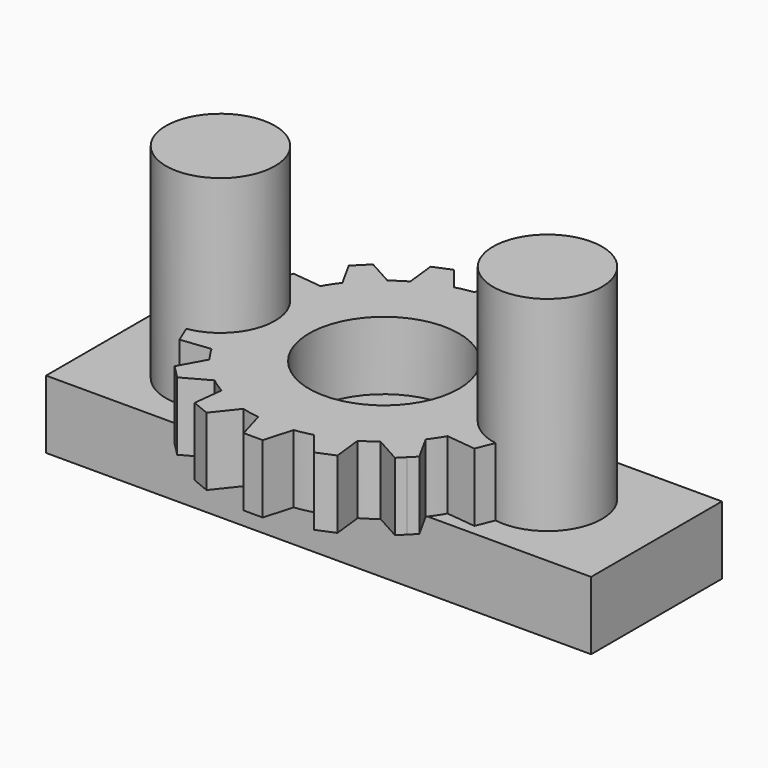
from build123d import *

# Parameters (mm, degrees)
F0_R     = 27.5
F1_DEPTH = 25
F2_W     = 200
F2_H     = 60
F2_R     = 20
F3_DEPTH = 25
F4_DEPTH = 75


with BuildPart() as f1:
    # F0 (on Top) → F1 (new body)
    with BuildSketch(Plane.XY):
        with BuildLine():
            ThreePointArc((-24.9770158815, 43.3145319454), (-19.1341716183, 46.1939766256), (-12.9665819589, 48.2894165662))
            Line((-12.9665819589, 48.2894165662), (-19.7274275781, 56.772163964))
            Line((-19.7274275781, 56.772163964), (-22.9610059419, 55.4327719507))
            Line((-22.9610059419, 55.4327719507), (-26.1945843057, 54.0933799374))
            Line((-26.1945843057, 54.0933799374), (-24.9770158815, 43.3145319454))
        make_face()
        with BuildLine():
            ThreePointArc((-39.6515075123, 30.4591193569), (-35.3553390593, 35.3553390593), (-30.4591193569, 39.6515075123))
            Line((-30.4591193569, 39.6515075123), (-39.951533137, 44.9012806053))
            Line((-39.951533137, 44.9012806053), (-42.4264068712, 42.4264068712))
            Line((-42.4264068712, 42.4264068712), (-44.9012806053, 39.951533137))
            Line((-44.9012806053, 39.951533137), (-39.6515075123, 30.4591193569))
        make_face()
        with BuildLine():
            ThreePointArc((-48.2894165662, 12.9665819589), (-46.1939766256, 19.1341716183), (-43.3145319454, 24.9770158815))
            Line((-43.3145319454, 24.9770158815), (-54.0933799374, 26.1945843057))
            Line((-54.0933799374, 26.1945843057), (-55.4327719507, 22.9610059419))
            Line((-55.4327719507, 22.9610059419), (-56.772163964, 19.7274275781))
            Line((-56.772163964, 19.7274275781), (-48.2894165662, 12.9665819589))
        make_face()
        with BuildLine():
            Line((-54.0933799374, -26.1945843057), (-43.3145319454, -24.9770158815))
            ThreePointArc((-43.3145319454, -24.9770158815), (-46.1939766256, -19.1341716183), (-48.2894165662, -12.9665819589))
            Line((-48.2894165662, -12.9665819589), (-56.772163964, -19.7274275781))
            Line((-56.772163964, -19.7274275781), (-55.4327719507, -22.9610059419))
            Line((-55.4327719507, -22.9610059419), (-54.0933799374, -26.1945843057))
        make_face()
        with BuildLine():
            Line((-39.951533137, -44.9012806053), (-30.4591193569, -39.6515075123))
            ThreePointArc((-30.4591193569, -39.6515075123), (-35.3553390593, -35.3553390593), (-39.6515075123, -30.4591193569))
            Line((-39.6515075123, -30.4591193569), (-44.9012806053, -39.951533137))
            Line((-44.9012806053, -39.951533137), (-42.4264068712, -42.4264068712))
            Line((-42.4264068712, -42.4264068712), (-39.951533137, -44.9012806053))
        make_face()
        with BuildLine():
            Line((-19.7274275781, -56.772163964), (-12.9665819589, -48.2894165662))
            ThreePointArc((-12.9665819589, -48.2894165662), (-19.1341716183, -46.1939766256), (-24.9770158815, -43.3145319454))
            Line((-24.9770158815, -43.3145319454), (-26.1945843057, -54.0933799374))
            Line((-26.1945843057, -54.0933799374), (-22.9610059419, -55.4327719507))
            Line((-22.9610059419, -55.4327719507), (-19.7274275781, -56.772163964))
        make_face()
        with BuildLine():
            Line((26.1945843057, -54.0933799374), (24.9770158815, -43.3145319454))
            ThreePointArc((24.9770158815, -43.3145319454), (19.1341716183, -46.1939766256), (12.9665819589, -48.2894165662))
            Line((12.9665819589, -48.2894165662), (19.7274275781, -56.772163964))
            Line((19.7274275781, -56.772163964), (22.9610059419, -55.4327719507))
            Line((22.9610059419, -55.4327719507), (26.1945843057, -54.0933799374))
        make_face()
        with BuildLine():
            Line((44.9012806053, -39.951533137), (39.6515075123, -30.4591193569))
            ThreePointArc((39.6515075123, -30.4591193569), (35.3553390593, -35.3553390593), (30.4591193569, -39.6515075123))
            Line((30.4591193569, -39.6515075123), (39.951533137, -44.9012806053))
            Line((39.951533137, -44.9012806053), (42.4264068712, -42.4264068712))
            Line((42.4264068712, -42.4264068712), (44.9012806053, -39.951533137))
        make_face()
        with BuildLine():
            Line((56.772163964, -19.7274275781), (48.2894165662, -12.9665819589))
            ThreePointArc((48.2894165662, -12.9665819589), (46.1939766256, -19.1341716183), (43.3145319454, -24.9770158815))
            Line((43.3145319454, -24.9770158815), (54.0933799374, -26.1945843057))
            Line((54.0933799374, -26.1945843057), (55.4327719507, -22.9610059419))
            Line((55.4327719507, -22.9610059419), (56.772163964, -19.7274275781))
        make_face()
        with BuildLine():
            ThreePointArc((49.5756996925, 6.5), (49.8938121646, 3.2569168991), (50, 0))
            ThreePointArc((50, 0), (49.8938121646, -3.2569168991), (49.5756996925, -6.5))
            Line((49.5756996925, -6.5), (60, -3.5))
            Line((60, -3.5), (60, 0))
            Line((60, 0), (60, 3.5))
            Line((60, 3.5), (49.5756996925, 6.5))
        make_face()
        with BuildLine():
            ThreePointArc((43.3145319454, 24.9770158815), (46.1939766256, 19.1341716183), (48.2894165662, 12.9665819589))
            Line((48.2894165662, 12.9665819589), (56.772163964, 19.7274275781))
            Line((56.772163964, 19.7274275781), (55.4327719507, 22.9610059419))
            Line((55.4327719507, 22.9610059419), (54.0933799374, 26.1945843057))
            Line((54.0933799374, 26.1945843057), (43.3145319454, 24.9770158815))
        make_face()
        with BuildLine():
            ThreePointArc((30.4591193569, 39.6515075123), (35.3553390593, 35.3553390593), (39.6515075123, 30.4591193569))
            Line((39.6515075123, 30.4591193569), (44.9012806053, 39.951533137))
            Line((44.9012806053, 39.951533137), (42.4264068712, 42.4264068712))
            Line((42.4264068712, 42.4264068712), (39.951533137, 44.9012806053))
            Line((39.951533137, 44.9012806053), (30.4591193569, 39.6515075123))
        make_face()
        with BuildLine():
            ThreePointArc((12.9665819589, 48.2894165662), (19.1341716183, 46.1939766256), (24.9770158815, 43.3145319454))
            Line((24.9770158815, 43.3145319454), (26.1945843057, 54.0933799374))
            Line((26.1945843057, 54.0933799374), (22.9610059419, 55.4327719507))
            Line((22.9610059419, 55.4327719507), (19.7274275781, 56.772163964))
            Line((19.7274275781, 56.772163964), (12.9665819589, 48.2894165662))
        make_face()
        with BuildLine():
            ThreePointArc((-6.5, 49.5756996925), (0, 50), (6.5, 49.5756996925))
            Line((6.5, 49.5756996925), (3.5, 60))
            Line((3.5, 60), (0, 60))
            Line((0, 60), (-3.5, 60))
            Line((-3.5, 60), (-6.5, 49.5756996925))
        make_face()
        with BuildLine():
            Line((3.5, -60), (6.5, -49.5756996925))
            ThreePointArc((6.5, -49.5756996925), (0, -50), (-6.5, -49.5756996925))
            Line((-6.5, -49.5756996925), (-3.5, -60))
            Line((-3.5, -60), (0, -60))
            Line((0, -60), (3.5, -60))
        make_face()
        with BuildLine():
            ThreePointArc((-49.5756996925, -6.5), (-50, 0), (-49.5756996925, 6.5))
            Line((-49.5756996925, 6.5), (-60, 3.5))
            Line((-60, 3.5), (-60, 0))
            Line((-60, 0), (-60, -3.5))
            Line((-60, -3.5), (-49.5756996925, -6.5))
        make_face()
        with BuildLine():
            ThreePointArc((49.5756996925, -6.5), (49.8938121646, -3.2569168991), (50, 0))
            ThreePointArc((50, 0), (49.8938121646, 3.2569168991), (49.5756996925, 6.5))
            ThreePointArc((49.5756996925, 6.5), (49.0392640202, 9.7545161008), (48.2894165662, 12.9665819589))
            ThreePointArc((48.2894165662, 12.9665819589), (46.1939766256, 19.1341716183), (43.3145319454, 24.9770158815))
            ThreePointArc((43.3145319454, 24.9770158815), (41.5734806151, 27.778511651), (39.6515075123, 30.4591193569))
            ThreePointArc((39.6515075123, 30.4591193569), (35.3553390593, 35.3553390593), (30.4591193569, 39.6515075123))
            ThreePointArc((30.4591193569, 39.6515075123), (27.778511651, 41.5734806151), (24.9770158815, 43.3145319454))
            ThreePointArc((24.9770158815, 43.3145319454), (19.1341716183, 46.1939766256), (12.9665819589, 48.2894165662))
            ThreePointArc((12.9665819589, 48.2894165662), (9.7545161008, 49.0392640202), (6.5, 49.5756996925))
            ThreePointArc((6.5, 49.5756996925), (0, 50), (-6.5, 49.5756996925))
            ThreePointArc((-6.5, 49.5756996925), (-9.7545161008, 49.0392640202), (-12.9665819589, 48.2894165662))
            ThreePointArc((-12.9665819589, 48.2894165662), (-19.1341716183, 46.1939766256), (-24.9770158815, 43.3145319454))
            ThreePointArc((-24.9770158815, 43.3145319454), (-27.778511651, 41.5734806151), (-30.4591193569, 39.6515075123))
            ThreePointArc((-30.4591193569, 39.6515075123), (-35.3553390593, 35.3553390593), (-39.6515075123, 30.4591193569))
            ThreePointArc((-39.6515075123, 30.4591193569), (-41.5734806151, 27.778511651), (-43.3145319454, 24.9770158815))
            ThreePointArc((-43.3145319454, 24.9770158815), (-46.1939766256, 19.1341716183), (-48.2894165662, 12.9665819589))
            ThreePointArc((-48.2894165662, 12.9665819589), (-49.0392640202, 9.7545161008), (-49.5756996925, 6.5))
            ThreePointArc((-49.5756996925, 6.5), (-50, 0), (-49.5756996925, -6.5))
            ThreePointArc((-49.5756996925, -6.5), (-49.0392640202, -9.7545161008), (-48.2894165662, -12.9665819589))
            ThreePointArc((-48.2894165662, -12.9665819589), (-46.1939766256, -19.1341716183), (-43.3145319454, -24.9770158815))
            ThreePointArc((-43.3145319454, -24.9770158815), (-41.5734806151, -27.778511651), (-39.6515075123, -30.4591193569))
            ThreePointArc((-39.6515075123, -30.4591193569), (-35.3553390593, -35.3553390593), (-30.4591193569, -39.6515075123))
            ThreePointArc((-30.4591193569, -39.6515075123), (-27.778511651, -41.5734806151), (-24.9770158815, -43.3145319454))
            ThreePointArc((-24.9770158815, -43.3145319454), (-19.1341716183, -46.1939766256), (-12.9665819589, -48.2894165662))
            ThreePointArc((-12.9665819589, -48.2894165662), (-9.7545161008, -49.0392640202), (-6.5, -49.5756996925))
            ThreePointArc((-6.5, -49.5756996925), (0, -50), (6.5, -49.5756996925))
            ThreePointArc((6.5, -49.5756996925), (9.7545161008, -49.0392640202), (12.9665819589, -48.2894165662))
            ThreePointArc((12.9665819589, -48.2894165662), (19.1341716183, -46.1939766256), (24.9770158815, -43.3145319454))
            ThreePointArc((24.9770158815, -43.3145319454), (27.778511651, -41.5734806151), (30.4591193569, -39.6515075123))
            ThreePointArc((30.4591193569, -39.6515075123), (35.3553390593, -35.3553390593), (39.6515075123, -30.4591193569))
            ThreePointArc((39.6515075123, -30.4591193569), (41.5734806151, -27.778511651), (43.3145319454, -24.9770158815))
            ThreePointArc((43.3145319454, -24.9770158815), (46.1939766256, -19.1341716183), (48.2894165662, -12.9665819589))
            ThreePointArc((48.2894165662, -12.9665819589), (49.0392640202, -9.7545161008), (49.5756996925, -6.5))
        make_face()
        Circle(F0_R, mode=Mode.SUBTRACT)
    extrude(amount=F1_DEPTH)


with BuildPart() as f3:
    # F2 (on Top) → F3 (new body)
    with BuildSketch(Plane.XY):
        Rectangle(F2_W, F2_H)
        with Locations((-60, 0)):
            Circle(F2_R, mode=Mode.SUBTRACT)
        with Locations((60, 0)):
            Circle(F2_R, mode=Mode.SUBTRACT)
        with Locations((-60, 0)):
            Circle(F2_R)
        with Locations((60, 0)):
            Circle(F2_R)
    extrude(amount=-F3_DEPTH)

    # F2 (on Top) → F4 (join)
    with BuildSketch(Plane.XY):
        with Locations((60, 0)):
            Circle(F2_R)
        with Locations((-60, 0)):
            Circle(F2_R)
    extrude(amount=F4_DEPTH)


solid = Compound([f1.part, f3.part])
